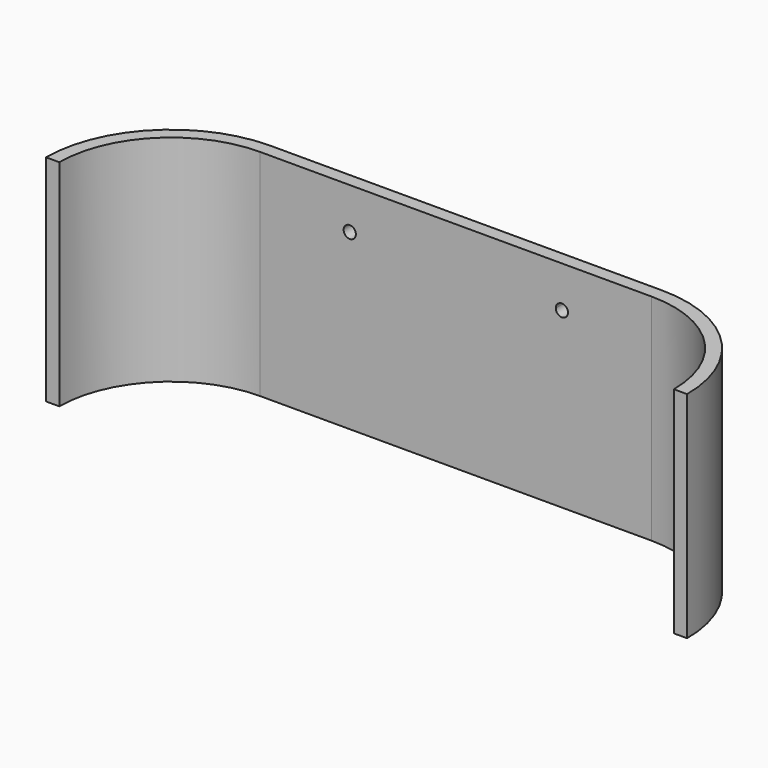
from build123d import *

# Parameters (mm, degrees)
F0_W     = 118.1
F0_H     = 60.85
F1_DEPTH = 2.5
F4_DEPTH = 32.925
F5_DEPTH = 30.425
F6_DEPTH = 2.5
F7_DEPTH = 1.5
F9_DEPTH = 25


# Not quite as in the source:
# - a feature of the source that left no trace in its solid (it failed there, or was rolled back) is left out
# - a pattern or mirror of a feature is missing from the dataset's text; its kind, count and spacing are read off the source's solid


with BuildPart() as f1:
    # F0 (on Front) → F1 (new body)
    with BuildSketch(Plane.XZ):
        Rectangle(F0_W, F0_H)
    extrude(amount=F1_DEPTH)

    # F1_copies: F1 across plane


with BuildPart() as f1_1:
    add(f1.part)
    add(f1.part.mirror(Plane.ZX.offset(-0.5)))

    # F3 (on Top) → F4 (join)
    with BuildSketch(Plane.XY):
        with BuildLine():
            ThreePointArc((-92.7, -36.15), (-82.8441431869, -12.3558568131), (-59.05, -2.5))
            Line((-59.05, -2.5), (-59.05, 0))
            Line((-59.05, 0), (-59.05, 1.5))
            ThreePointArc((-59.05, 1.5), (-85.6725703117, -9.5274296883), (-96.7, -36.15))
            Line((-96.7, -36.15), (-95.2, -36.15))
            Line((-95.2, -36.15), (-92.7, -36.15))
        make_face()
        with BuildLine():
            ThreePointArc((59.05, -2.5), (82.8441431869, -12.3558568131), (92.7, -36.15))
            Line((92.7, -36.15), (95.2, -36.15))
            Line((95.2, -36.15), (96.7, -36.15))
            ThreePointArc((96.7, -36.15), (85.6725703117, -9.5274296883), (59.05, 1.5))
            Line((59.05, 1.5), (59.05, 0))
            Line((59.05, 0), (59.05, -2.5))
        make_face()
    extrude(amount=F4_DEPTH)

    # F3 (on Top) → F5 (join)
    with BuildSketch(Plane.XY):
        with BuildLine():
            ThreePointArc((-92.7, -36.15), (-82.8441431869, -12.3558568131), (-59.05, -2.5))
            Line((-59.05, -2.5), (-59.05, 0))
            Line((-59.05, 0), (-59.05, 1.5))
            ThreePointArc((-59.05, 1.5), (-85.6725703117, -9.5274296883), (-96.7, -36.15))
            Line((-96.7, -36.15), (-95.2, -36.15))
            Line((-95.2, -36.15), (-92.7, -36.15))
        make_face()
        with BuildLine():
            ThreePointArc((59.05, -2.5), (82.8441431869, -12.3558568131), (92.7, -36.15))
            Line((92.7, -36.15), (95.2, -36.15))
            Line((95.2, -36.15), (96.7, -36.15))
            ThreePointArc((96.7, -36.15), (85.6725703117, -9.5274296883), (59.05, 1.5))
            Line((59.05, 1.5), (59.05, 0))
            Line((59.05, 0), (59.05, -2.5))
        make_face()
    extrude(amount=-F5_DEPTH)

    # F6 (add): a face of the model
    f6_faces = [f1_1.faces().sort_by_distance(p)[0] for p in [
        (0, -0.5, 30.425),
    ]]
    extrude(f6_faces, amount=F6_DEPTH)

    # F7 (add): a face of the model
    f7_faces = [f1_1.faces().sort_by_distance(p)[0] for p in [
        (84.2373603721, -10.9626396279, 32.925),
    ]]
    extrude(f7_faces, amount=F7_DEPTH)

    # F8 (on face) → F9 (cut)
    with BuildSketch(Plane(origin=(0, 1.5, 0), x_dir=(-1, 0, 0), z_dir=(0, 1, 0))):
        with BuildLine():
            ThreePointArc((33.85, 21.945), (32, 23.795), (30.15, 21.945))
            ThreePointArc((30.15, 21.945), (32, 20.095), (33.85, 21.945))
        make_face()
        with BuildLine():
            ThreePointArc((-32, 23.795), (-33.3081475452, 20.6368524548), (-30.15, 21.945))
            ThreePointArc((-30.15, 21.945), (-30.6918524548, 23.2531475452), (-32, 23.795))
        make_face()
    extrude(amount=-F9_DEPTH, mode=Mode.SUBTRACT)


solid = f1_1.part
